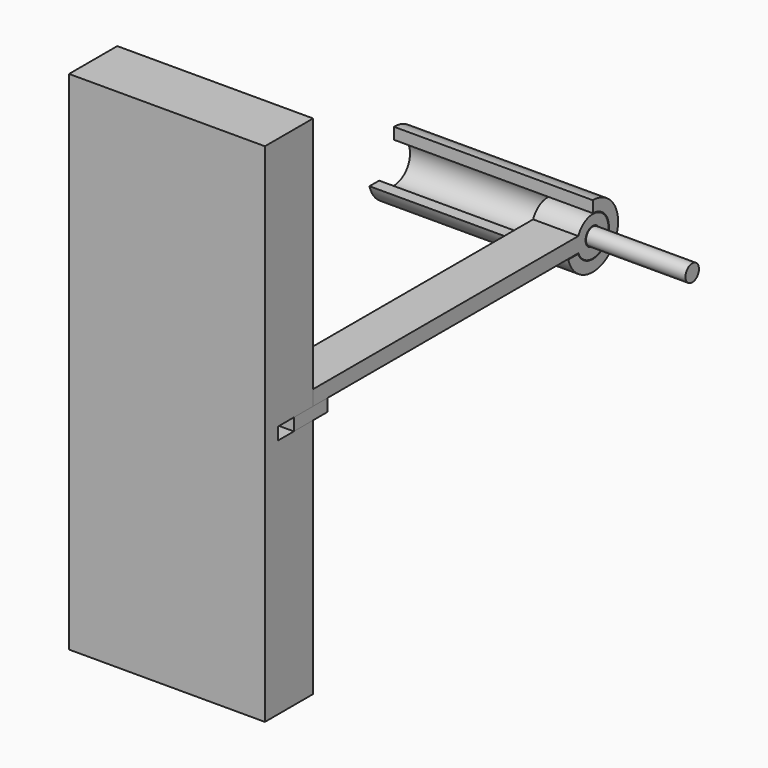
from build123d import *

# Parameters (mm, degrees)
F0_W      = 7.5
F0_H      = 55
F1_DEPTH  = 2.5
F2_R      = 1.5
F3_DEPTH  = 7.5
F5_DEPTH  = 33
F2_R_2    = 1.4010319541
F6_DEPTH  = 16.5
F9_DEPTH  = 7.5
F11_DEPTH = 32.5


# Not quite as in the source:
# - ends of sketch curves that miss each other by under 0.0002 mm in the source are joined
# - the program builds the solid bodies; features that only make, move or delete a surface that nothing else refers to are left out


with BuildPart() as f1:
    # F0 (on Top) → F1 (new body)
    with BuildSketch(Plane.XY):
        with Locations((11.75, -27.5)):
            Rectangle(F0_W, F0_H)
    extrude(amount=F1_DEPTH)

    # F2 (on face) → F3 (join)
    with BuildSketch(Plane.YZ.offset(15.5)):
        with BuildLine():
            ThreePointArc((0, 0), (6.2500474018, 1.249781204), (8.07847e-05, 2.4999663372))
            Line((8.07847e-05, 2.4999663372), (0, 2.4997724509))
            Line((0, 2.4997724509), (0, 0))
        make_face()
        with Locations((3.0000474035, 1.2689229439)):
            Circle(F2_R, mode=Mode.SUBTRACT)
    extrude(amount=-F3_DEPTH)


with BuildPart() as f5:
    # F2 (on face) → F5 (new body)
    with BuildSketch(Plane.YZ.offset(15.5)):
        with BuildLine():
            Line((-0.0574924529, -0.1), (-2.0730679938, -0.1))
            ThreePointArc((-2.0730679938, -0.1), (7.1715905231, -1.926179224), (3.0000474035, 6.5234876129))
            Line((3.0000474035, 6.5234876129), (3.0000474035, 4.6189229439))
            ThreePointArc((3.0000474035, 4.6189229439), (5.8114875916, -0.552698331), (-0.0574924529, -0.1))
        make_face()
    extrude(amount=-F5_DEPTH)


with BuildPart() as f6:
    # F2 (on face) → F6 (new body)
    with BuildSketch(Plane.YZ.offset(15.5)):
        with Locations((3.0000474035, 1.2689229439)):
            Circle(F2_R_2)
    extrude(amount=F6_DEPTH)


with BuildPart() as f9:
    # F8 (on face) → F9 (new body)
    with BuildSketch(Plane.YZ.offset(15.5)):
        Polygon((-52, -2.0469013694), (-52, 0), (-55, 0), (-59, 0), (-59, -2.0469013694), align=None)
    extrude(amount=-F9_DEPTH)


with BuildPart() as f11:
    # F10 (on face) → F11 (new body)
    with BuildSketch(Plane.YZ.offset(15.5)):
        Polygon((-59, 0), (-55.021867156, 0), (-54.99, 0), (-55.0059096515, 2.0469013694), (-55.0059096515, 42.0469013694), (-65.0059096515, 42.0469013694), (-65.0059096515, 2.0470365488), (-65.0059096515, 0), (-65.0059096515, -2.0470365488), (-65.0059096515, -42.0469013694), (-55.0059096515, -42.0469013694), (-55.0059096515, -2.0469013694), (-55.021867156, -2.0469013694), (-58.9999999993, -2.0469553613), (-62.3021833599, -2.047), (-62.3021833599, 0), align=None)
    extrude(amount=-F11_DEPTH)


solid = Compound([f1.part, f5.part, f6.part, f9.part, f11.part])
